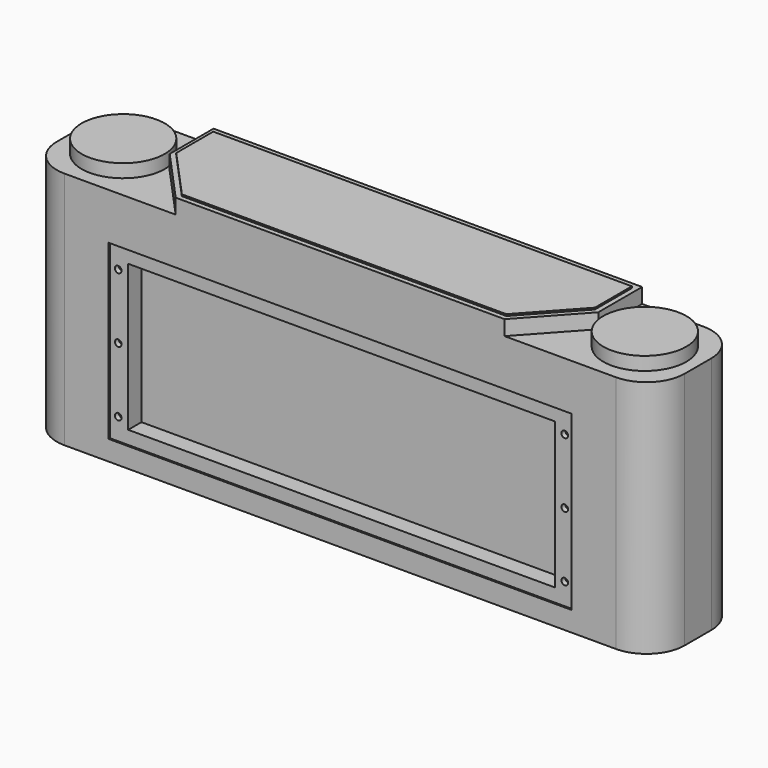
from build123d import *

# Parameters (mm, degrees)
F1_DEPTH  = 33
F3_DEPTH  = 5
F4_R      = 12.5
F5_DEPTH  = 4
F7_DEPTH  = 0.5
F8_R      = 11.5
F9_R      = 11.5
F11_DEPTH = 0.5
F13_DEPTH = 5
F12_R     = 1
F14_DEPTH = 1.5
F15_ANGLE = 180


with BuildPart() as f1:
    # F0 (on Front) → F1 (new body)
    with BuildSketch(Plane.XZ):
        Polygon((64.5, 38.5), (0, 38.5), (-64.5, 38.5), (-94.5, 38.5), (-94.5, 0), (-94.5, -38.5), (0, -38.5), (94.5, -38.5), (94.5, 0), (94.5, 38.5), align=None)
    extrude(amount=F1_DEPTH)

    # F2 (on face) → F3 (cut)
    with BuildSketch(Plane.XY.offset(38.5)):
        Polygon((-64.5, 0), (-94.5, 0), (-94.5, -16.5), (-94.5, -33), (-64.5, -33), (-64.5, -16.5), (-49.5, 0), align=None)
        Polygon((49.5, 0), (64.5, -16.5), (64.5, -33), (94.5, -33), (94.5, 0), (64.5, 0), align=None)
    extrude(amount=-F3_DEPTH, mode=Mode.SUBTRACT)

    # F4 (on face) → F5 (join)
    with BuildSketch(Plane.XY.offset(33.5)):
        with BuildLine():
            ThreePointArc((-66, -16.5), (-78.5, -4), (-91, -16.5))
            ThreePointArc((-91, -16.5), (-78.5, -29), (-66, -16.5))
        make_face()
        with Locations((78.5, -16.5)):
            Circle(F4_R)
    extrude(amount=F5_DEPTH)

    # F6 (on face) → F7 (cut)
    with BuildSketch(Plane.XY.offset(38.5)):
        Polygon((0, -1.5), (0, 0), (-49.5, 0), (-64.5, -16.5), (-64.5, -33), (0, -33), (0, -31), (-63, -31), (-63, -17.0799103121), (-48.8364451708, -1.5), align=None)
        Polygon((49.5, 0), (0, 0), (0, -1.5), (48.8364451708, -1.5), (63, -17.0799103121), (63, -31), (0, -31), (0, -33), (64.5, -33), (64.5, -16.5), align=None)
    extrude(amount=-F7_DEPTH, mode=Mode.SUBTRACT)

    # F8
    f8_edges = [f1.edges().sort_by_distance(p)[0] for p in [
        (-94.5, -33, -2.5),
    ]]
    fillet(f8_edges, radius=F8_R)

    # F9
    f9_edges = [f1.edges().sort_by_distance(p)[0] for p in [
        (-94.5, 0, -2.5),
        (94.5, 0, -2.5),
        (94.5, -33, -2.5),
    ]]
    fillet(f9_edges, radius=F9_R)

    # F10 (on Front) → F11 (cut)
    with BuildSketch(Plane.XZ):
        Polygon((69.7, -32.5), (69.7, 0), (69.7, 19.5), (0, 19.5), (-69.7, 19.5), (-69.7, 0), (-69.7, -32.5), (0, -32.5), align=None)
    extrude(amount=F11_DEPTH, mode=Mode.SUBTRACT)

    # F12 (on face) → F13 (cut)
    with BuildSketch(Plane(origin=(0, -0.5, 0), x_dir=(-1, 0, 0), z_dir=(0, 1, 0))):
        Polygon((-64.2, 15.5), (-64.2, 0), (-64.2, -28.5), (-48.5950261354, -28.5), (64.2, -28.5), (64.2, 15.5), (-38.0094833672, 15.5), align=None)
    extrude(amount=-F13_DEPTH, mode=Mode.SUBTRACT)

    # F12 (on face) → F14 (cut)
    with BuildSketch(Plane(origin=(0, -0.5, 0), x_dir=(-1, 0, 0), z_dir=(0, 1, 0))):
        with BuildLine():
            ThreePointArc((-66.2, 13), (-66.4928932188, 13.7071067812), (-67.2, 14))
            ThreePointArc((-67.2, 14), (-67.9071067812, 12.2928932188), (-66.2, 13))
        make_face()
        with BuildLine():
            ThreePointArc((-66.2, -6.5), (-66.4928932188, -5.7928932188), (-67.2, -5.5))
            ThreePointArc((-67.2, -5.5), (-67.9071067812, -7.2071067812), (-66.2, -6.5))
        make_face()
        with Locations((67.2, -26)):
            Circle(F12_R)
        with Locations((67.2, -6.5)):
            Circle(F12_R)
        with Locations((67.2, 13)):
            Circle(F12_R)
        with BuildLine():
            ThreePointArc((-66.2, -26), (-67.9071067812, -25.2928932188), (-67.2, -27))
            ThreePointArc((-67.2, -27), (-66.4928932188, -26.7071067812), (-66.2, -26))
        make_face()
    extrude(amount=-F14_DEPTH, mode=Mode.SUBTRACT)


with BuildPart() as f1_1:
    # F15: moved
    add(f1.part.rotate(Axis((83, 0, -2.5), (0, 0, 1)), F15_ANGLE))


with BuildPart() as f1_2:
    # F16: moved
    add(f1_1.part.moved(Location((-166, 0, 0))))


solid = f1_2.part
